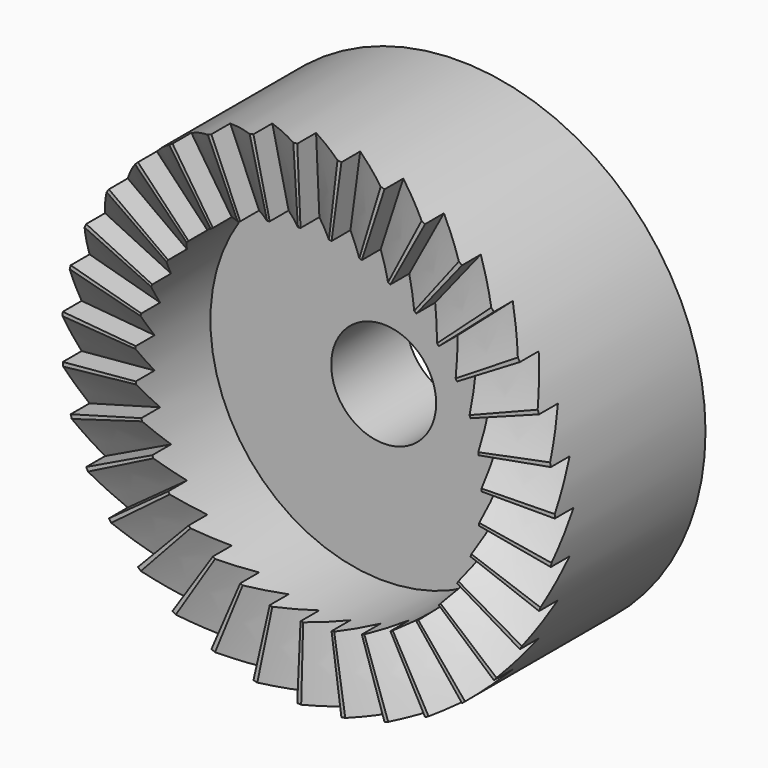
from build123d import *

# Parameters (mm, degrees)
F0_R            = 66.4533293616
F1_DEPTH        = 25.4
F2_R            = 66.4533293616
F2_R_2          = 46.7097239964
F3_DEPTH        = 25.4
F4_R            = 14.1472200922
F5_DEPTH        = 25.401
F9_COPIES_COUNT = 35


# Not quite as in the source:
# - a pattern or mirror of a feature is missing from the dataset's text; its kind, count and spacing are read off the source's solid


with BuildPart() as f1:
    # F0 (on Front) → F1 (new body)
    with BuildSketch(Plane.XZ):
        Circle(F0_R)
    extrude(amount=F1_DEPTH)

    # F2 (on face) → F3 (join)
    with BuildSketch(Plane.XZ.offset(25.4)):
        Circle(F2_R)
        Circle(F2_R_2, mode=Mode.SUBTRACT)
    extrude(amount=F3_DEPTH)

    # F4 (on face) → F5 (cut, through all)
    with BuildSketch(Plane.XZ.offset(25.4)):
        Circle(F4_R)
    extrude(amount=-F5_DEPTH, mode=Mode.SUBTRACT)

    # F6 (on Right) → F9 section 0
    with BuildSketch(Plane.YZ):
        Polygon((-50.8, -0.1108396623), (-44.45, 0), (-50.8, 0), align=None)
    # F8 (on offset) → F9 section 1
    with BuildSketch(Plane.YZ.offset(66.675)):
        Polygon((-50.8, -10.9985226281), (-44.45, 0), (-50.8, 0), align=None)
    f9 = loft(mode=Mode.SUBTRACT)

    # F9_copies: F9 ×35 about axis
    f9_copies_axis = Axis((0, 0, 0), (0, 1, 0))
    for i in range(1, F9_COPIES_COUNT):
        add(f9.rotate(f9_copies_axis, i * 360 / F9_COPIES_COUNT), mode=Mode.SUBTRACT)


solid = f1.part
